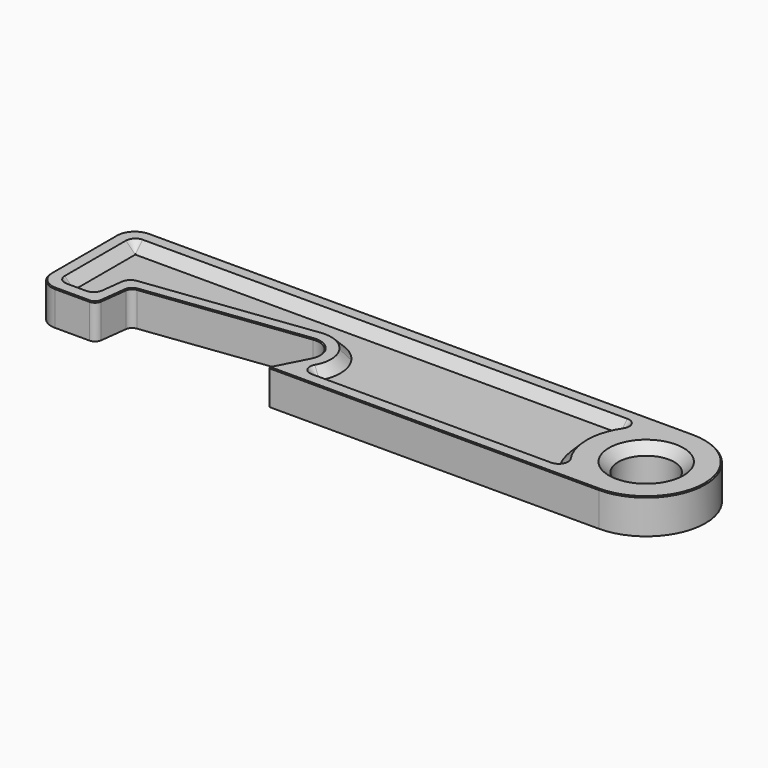
from build123d import *

# Parameters (mm, degrees)
F0_R     = 6
F1_DEPTH = 7.5
F3_DEPTH = 2
F4_SIZE  = 1.99999
F5_SIZE  = 2
F6_SIZE  = 0.2


# Not quite as in the source:
# - a fillet or chamfer is up to 0.001 mm smaller than in the source, because OpenCascade refuses the exact size


with BuildPart() as f1:
    # F0 (on Top) → F1 (new body)
    with BuildSketch(Plane.XY):
        with BuildLine():
            Line((0, 12.7), (-116.65, 12.7))
            ThreePointArc((-116.65, 12.7), (-119.4784271247, 11.5284271247), (-120.65, 8.7))
            Line((-120.65, 8.7), (-120.65, -8.7))
            ThreePointArc((-120.65, -8.7), (-119.4784271247, -11.5284271247), (-116.65, -12.7))
            Line((-116.65, -12.7), (-109.2756163486, -12.7))
            ThreePointArc((-109.2756163486, -12.7), (-108.2823049478, -12.323980632), (-107.7869993139, -11.3844432814))
            Line((-107.7869993139, -11.3844432814), (-107.0773577752, -5.6570214144))
            ThreePointArc((-107.0773577752, -5.6570214144), (-106.6508978642, -4.7823035915), (-105.77738814, -4.3533745914))
            Line((-105.77738814, -4.3533745914), (-71.4370597318, 0))
            ThreePointArc((-71.4370597318, 0), (-68.2894054117, -0.967220541), (-66.934, -3.9682402783))
            ThreePointArc((-66.934, -3.9682402783), (-67.0466854589, -4.910994572), (-67.3783928291, -5.8006315156))
            Line((-67.3783928291, -5.8006315156), (-70.7461413924, -12.3354755477))
            ThreePointArc((-70.7461413924, -12.3354755477), (-70.7373768459, -12.5801324074), (-70.5239159442, -12.7))
            Line((-70.5239159442, -12.7), (0, -12.7))
            ThreePointArc((0, -12.7), (12.7, 0), (0, 12.7))
        make_face()
        Circle(F0_R, mode=Mode.SUBTRACT)
    extrude(amount=F1_DEPTH)

    # F2 (on face) → F3 (cut)
    with BuildSketch(Plane.XY.offset(7.5)):
        with BuildLine():
            ThreePointArc((-10.5404901245, -7.0843537415), (-12.7, 0), (-10.5404901245, 7.0843537415))
            ThreePointArc((-10.5404901245, 7.0843537415), (-10.4352904965, 9.1404008409), (-12.2004098292, 10.2))
            Line((-12.2004098292, 10.2), (-116.15, 10.2))
            ThreePointArc((-116.15, 10.2), (-117.5642135624, 9.6142135624), (-118.15, 8.2))
            Line((-118.15, 8.2), (-118.15, -8.2))
            ThreePointArc((-118.15, -8.2), (-117.5642135624, -9.6142135624), (-116.15, -10.2))
            Line((-116.15, -10.2), (-111.9268490457, -10.2))
            ThreePointArc((-111.9268490457, -10.2), (-110.6024338446, -9.6986408426), (-109.9420263328, -8.4459243752))
            Line((-109.9420263328, -8.4459243752), (-109.3672424661, -3.8069207262))
            ThreePointArc((-109.3672424661, -3.8069207262), (-108.7986292513, -2.6406302958), (-107.6339496191, -2.0687249623))
            Line((-107.6339496191, -2.0687249623), (-71.7514720642, 2.4801501739))
            ThreePointArc((-71.7514720642, 2.4801501739), (-68.3008484478, 1.9745295223), (-65.6082269333, -0.2418289696))
            ThreePointArc((-65.6082269333, -0.2418289696), (-64.4404924053, -3.6777938671), (-65.2968047441, -7.2042918302))
            ThreePointArc((-65.2968047441, -7.2042918302), (-65.2930945463, -9.2021436175), (-63.5622831269, -10.2))
            Line((-63.5622831269, -10.2), (-12.2004098292, -10.2))
            ThreePointArc((-12.2004098292, -10.2), (-10.4352904965, -9.1404008409), (-10.5404901245, -7.0843537415))
        make_face()
    extrude(amount=-F3_DEPTH, mode=Mode.SUBTRACT)

    # F4 (size 2 in the source; OpenCascade refuses exactly that, so slightly less here)
    f4_edges = [f1.edges().sort_by_distance(p)[0] for p in [
        (-12.7, 0, 5.5),
        (-10.43529, 9.140401, 5.5),
        (-64.175205, 10.2, 5.5),
        (-117.564214, 9.614214, 5.5),
        (-118.15, 0, 5.5),
        (-117.564214, -9.614214, 5.5),
        (-114.038425, -10.2, 5.5),
        (-110.602434, -9.698641, 5.5),
        (-109.654634, -6.126423, 5.5),
        (-108.798629, -2.64063, 5.5),
        (-89.692711, 0.205713, 5.5),
        (-65.525254, -0.363318, 5.5),
        (-65.293095, -9.202144, 5.5),
        (-37.881346, -10.2, 5.5),
        (-10.43529, -9.140401, 5.5),
    ]]
    chamfer(f4_edges, length=F4_SIZE)

    # F5
    f5_edges = [f1.edges().sort_by_distance(p)[0] for p in [
        (-6, 0, 7.5),
    ]]
    chamfer(f5_edges, length=F5_SIZE)

    # F6
    f6_edges = [f1.edges().sort_by_distance(p)[0] for p in [
        (-58.325, 12.7, 7.5),
    ]]
    chamfer(f6_edges, length=F6_SIZE)


solid = f1.part
